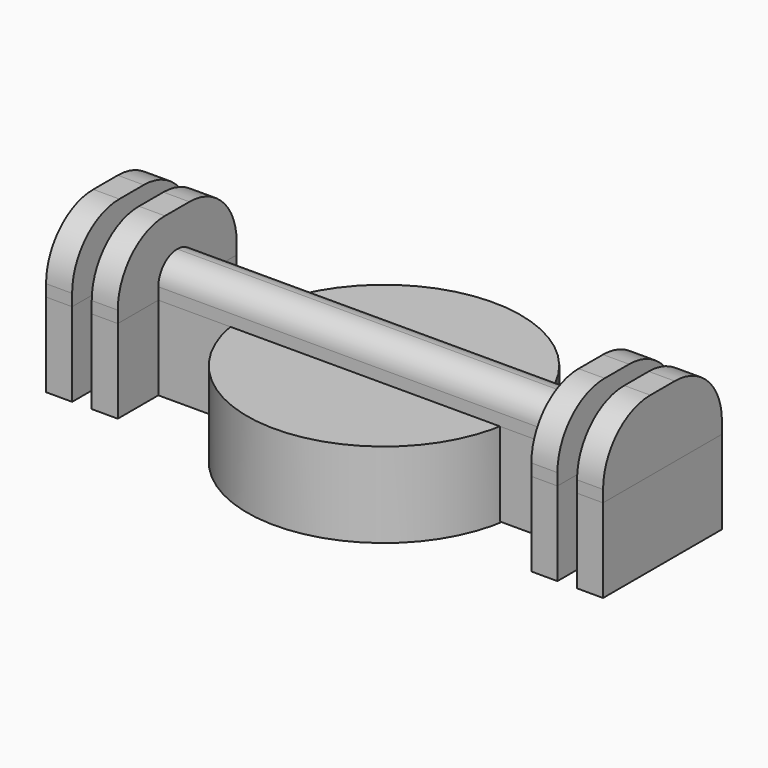
from build123d import *

# Parameters (mm, degrees)
F0_R     = 11.6
F0_R_2   = 9.6
F1_DEPTH = 5.2
F2_R     = 11.6
F2_R_2   = 9.6
F3_DEPTH = 2
F4_W     = 2.2083204985
F4_H     = 4
F4_H_2   = 4.2943226658
F4_W_2   = 1.1041602492
F4_W_3   = 1.6607893258
F5_DEPTH = 7.1
F6_DEPTH = 3
F7_DEPTH = 6
F8_R     = 5
F8_2_R   = 5
F8_3_R   = 5
F8_4_R   = 5
F9_R     = 1.99999
F9_2_R   = 1.99999
F9_3_R   = 1.99999


# Not quite as in the source:
# - a fillet or chamfer is up to 0.001 mm smaller than in the source, because OpenCascade refuses the exact size


with BuildPart() as f1:
    # F0 (on Top) → F1 (new body)
    with BuildSketch(Plane.XY):
        Circle(F0_R)
        Circle(F0_R_2, mode=Mode.SUBTRACT)
    extrude(amount=F1_DEPTH)

    # F2 (on face) → F3 (join)
    with BuildSketch(Plane.XY.offset(5.2)):
        Circle(F2_R)
        Circle(F2_R_2, mode=Mode.SUBTRACT)
        Circle(F2_R_2)
    extrude(amount=F3_DEPTH)


with BuildPart() as f5:
    # F4 (on face) → F5 (new body)
    with BuildSketch(Plane.XY.offset(7.2)):
        with BuildLine():
            Line((-11.4262854857, 2), (-17.5267299265, 2))
            Line((-17.5267299265, 2), (-17.5267299265, -2))
            Line((-17.5267299265, -2), (-11.4262854857, -2))
            ThreePointArc((-11.4262854857, -2), (-11.6, 0), (-11.4262854857, 2))
        make_face()
        with Locations((-18.6308901757, 0)):
            Rectangle(F4_W, F4_H)
        with Locations((-18.6308901757, -4.1471613329)):
            Rectangle(F4_W, F4_H_2)
        Polygon((-22.5, -2), (-22.5, 2), (-21.3958397508, 2), (-21.3958397508, 6.2943226658), (-23.6041602492, 6.2943226658), (-23.6041602492, -6.2943226658), (-21.3958397508, -6.2943226658), (-21.3958397508, -2), align=None)
        with Locations((-21.9479198754, 0)):
            Rectangle(F4_W_2, F4_H)
        with Locations((-18.6308901757, 4.1471613329)):
            Rectangle(F4_W, F4_H_2)
        with Locations((-20.5654450879, 0)):
            Rectangle(F4_W_3, F4_H)
    extrude(amount=-F5_DEPTH)


with BuildPart() as f5b:
    # F4 (on face) → F5, piece 2 (new body)
    with BuildSketch(Plane.XY.offset(7.2)):
        with BuildLine():
            Line((17.5267299265, 2), (11.4262854857, 2))
            ThreePointArc((11.4262854857, 2), (11.5564897706, 1.0037650039), (11.6, 0))
            ThreePointArc((11.6, 0), (11.5564897706, -1.0037650039), (11.4262854857, -2))
            Line((11.4262854857, -2), (17.5267299265, -2))
            Line((17.5267299265, -2), (17.5267299265, 2))
        make_face()
        with Locations((18.6308901757, 0)):
            Rectangle(F4_W, F4_H)
        with Locations((18.6308901757, -4.1471613329)):
            Rectangle(F4_W, F4_H_2)
        Polygon((21.3958397508, 6.2943226658), (21.3958397508, 2), (22.5, 2), (22.5, -2), (21.3958397508, -2), (21.3958397508, -6.2943226658), (23.6041602492, -6.2943226658), (23.6041602492, 6.2943226658), align=None)
        with Locations((20.5654450879, 0)):
            Rectangle(F4_W_3, F4_H)
        with Locations((18.6308901757, 4.1471613329)):
            Rectangle(F4_W, F4_H_2)
        with Locations((21.9479198754, 0)):
            Rectangle(F4_W_2, F4_H)
    extrude(amount=-F5_DEPTH)


with BuildPart() as f6:
    # F4 (on face) → F6 (new body)
    with BuildSketch(Plane.XY.offset(7.2)):
        with BuildLine():
            Line((-11.4262854857, 2), (-17.5267299265, 2))
            Line((-17.5267299265, 2), (-17.5267299265, -2))
            Line((-17.5267299265, -2), (-11.4262854857, -2))
            ThreePointArc((-11.4262854857, -2), (-11.6, 0), (-11.4262854857, 2))
        make_face()
        with BuildLine():
            Line((11.4262854857, 2), (-11.4262854857, 2))
            ThreePointArc((-11.4262854857, 2), (-11.6, 0), (-11.4262854857, -2))
            Line((-11.4262854857, -2), (11.4262854857, -2))
            ThreePointArc((11.4262854857, -2), (11.5564897706, -1.0037650039), (11.6, 0))
            ThreePointArc((11.6, 0), (11.5564897706, 1.0037650039), (11.4262854857, 2))
        make_face()
        with BuildLine():
            Line((17.5267299265, 2), (11.4262854857, 2))
            ThreePointArc((11.4262854857, 2), (11.5564897706, 1.0037650039), (11.6, 0))
            ThreePointArc((11.6, 0), (11.5564897706, -1.0037650039), (11.4262854857, -2))
            Line((11.4262854857, -2), (17.5267299265, -2))
            Line((17.5267299265, -2), (17.5267299265, 2))
        make_face()
    extrude(amount=F6_DEPTH)

    # F9 (radius 2 in the source; OpenCascade refuses exactly that, so slightly less here)
    f9_edges = [f6.edges().sort_by_distance(p)[0] for p in [
        (0, -2, 10.2),
        (0, 2, 10.2),
    ]]
    fillet(f9_edges, radius=F9_R)


with BuildPart() as f6b:
    # F4 (on face) → F6, piece 2 (new body)
    with BuildSketch(Plane.XY.offset(7.2)):
        with Locations((-20.5654450879, 0)):
            Rectangle(F4_W_3, F4_H)
    extrude(amount=F6_DEPTH)

    # F9#3 (radius 2 in the source; OpenCascade refuses exactly that, so slightly less here)
    f9_3_edges = [f6b.edges().sort_by_distance(p)[0] for p in [
        (-20.565445, -2, 10.2),
        (-20.565445, 2, 10.2),
    ]]
    fillet(f9_3_edges, radius=F9_3_R)


with BuildPart() as f6c:
    # F4 (on face) → F6, piece 3 (new body)
    with BuildSketch(Plane.XY.offset(7.2)):
        with Locations((20.5654450879, 0)):
            Rectangle(F4_W_3, F4_H)
    extrude(amount=F6_DEPTH)

    # F9#2 (radius 2 in the source; OpenCascade refuses exactly that, so slightly less here)
    f9_2_edges = [f6c.edges().sort_by_distance(p)[0] for p in [
        (20.565445, -2, 10.2),
        (20.565445, 2, 10.2),
    ]]
    fillet(f9_2_edges, radius=F9_2_R)


with BuildPart() as f7:
    # F4 (on face) → F7 (new body)
    with BuildSketch(Plane.XY.offset(7.2)):
        Polygon((-22.5, -2), (-22.5, 2), (-21.3958397508, 2), (-21.3958397508, 6.2943226658), (-23.6041602492, 6.2943226658), (-23.6041602492, -6.2943226658), (-21.3958397508, -6.2943226658), (-21.3958397508, -2), align=None)
        with Locations((-21.9479198754, 0)):
            Rectangle(F4_W_2, F4_H)
    extrude(amount=F7_DEPTH)

    # F8
    f8_edges = [f7.edges().sort_by_distance(p)[0] for p in [
        (-22.5, 6.294323, 13.2),
        (-22.5, -6.294323, 13.2),
    ]]
    fillet(f8_edges, radius=F8_R)


with BuildPart() as f7b:
    # F4 (on face) → F7, piece 2 (new body)
    with BuildSketch(Plane.XY.offset(7.2)):
        with Locations((-18.6308901757, 4.1471613329)):
            Rectangle(F4_W, F4_H_2)
        with Locations((-18.6308901757, 0)):
            Rectangle(F4_W, F4_H)
        with Locations((-18.6308901757, -4.1471613329)):
            Rectangle(F4_W, F4_H_2)
    extrude(amount=F7_DEPTH)

    # F8#2
    f8_2_edges = [f7b.edges().sort_by_distance(p)[0] for p in [
        (-18.63089, 6.294323, 13.2),
        (-18.63089, -6.294323, 13.2),
    ]]
    fillet(f8_2_edges, radius=F8_2_R)


with BuildPart() as f7c:
    # F4 (on face) → F7, piece 3 (new body)
    with BuildSketch(Plane.XY.offset(7.2)):
        with Locations((18.6308901757, 4.1471613329)):
            Rectangle(F4_W, F4_H_2)
        with Locations((18.6308901757, 0)):
            Rectangle(F4_W, F4_H)
        with Locations((18.6308901757, -4.1471613329)):
            Rectangle(F4_W, F4_H_2)
    extrude(amount=F7_DEPTH)

    # F8#3
    f8_3_edges = [f7c.edges().sort_by_distance(p)[0] for p in [
        (18.63089, -6.294323, 13.2),
        (18.63089, 6.294323, 13.2),
    ]]
    fillet(f8_3_edges, radius=F8_3_R)


with BuildPart() as f7d:
    # F4 (on face) → F7, piece 4 (new body)
    with BuildSketch(Plane.XY.offset(7.2)):
        Polygon((21.3958397508, 6.2943226658), (21.3958397508, 2), (22.5, 2), (22.5, -2), (21.3958397508, -2), (21.3958397508, -6.2943226658), (23.6041602492, -6.2943226658), (23.6041602492, 6.2943226658), align=None)
        with Locations((21.9479198754, 0)):
            Rectangle(F4_W_2, F4_H)
    extrude(amount=F7_DEPTH)

    # F8#4
    f8_4_edges = [f7d.edges().sort_by_distance(p)[0] for p in [
        (22.5, -6.294323, 13.2),
        (22.5, 6.294323, 13.2),
    ]]
    fillet(f8_4_edges, radius=F8_4_R)


solid = Compound([f1.part, f5.part, f5b.part, f6.part, f6b.part, f6c.part, f7.part, f7b.part, f7c.part, f7d.part])
